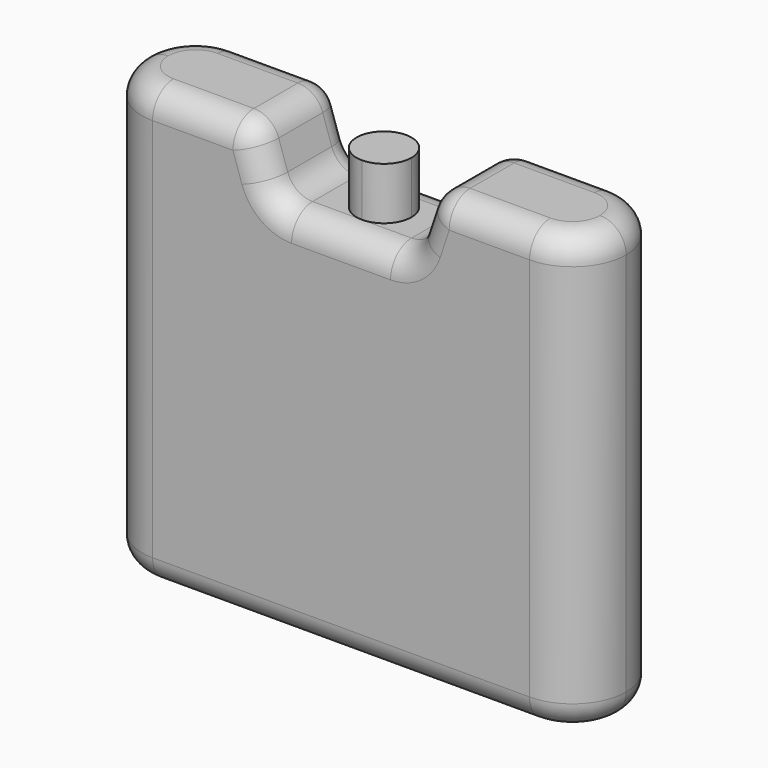
from build123d import *

# Parameters (mm, degrees)
F1_DEPTH = 20.5
F2_R     = 10.24999
F3_F1_R  = 5
F3_F2_R  = 5
F5_DEPTH = 10


# Not quite as in the source:
# - a fillet or chamfer is up to 0.001 mm smaller than in the source, because OpenCascade refuses the exact size


with BuildPart() as f1:
    # F0 (on Front) → F1 (new body)
    with BuildSketch(Plane.XZ):
        Polygon((0, 83.5), (0, 0), (46.25, 0), (46.25, 71.5), (33.2, 71.5), (29.2, 83.5), align=None)
        Polygon((46.25, 71.5), (46.25, 0), (92.5, 0), (92.5, 83.5), (63.3, 83.5), (59.3, 71.5), align=None)
    extrude(amount=F1_DEPTH)

    # F2 (radius 10.25 in the source; OpenCascade refuses exactly that, so slightly less here)
    f2_edges = [f1.edges().sort_by_distance(p)[0] for p in [
        (0, -20.5, 41.75),
        (0, 0, 41.75),
        (92.5, -20.5, 41.75),
        (92.5, 0, 41.75),
    ]]
    fillet(f2_edges, radius=F2_R)

    # F3: fillet of radius 5 on 24 edges, made by hand

    # F3_f1
    f3_f1_edges = [f1.edges().sort_by_distance(p)[0] for p in [
        (59.3, -10.25, 71.5),
        (33.2, -10.25, 71.5),
    ]]
    fillet(f3_f1_edges, radius=F3_F1_R)

    # F3_f2
    f3_f2_edges = [f1.edges().sort_by_distance(p)[0] for p in [
        (92.5, -10.25, 83.5),
        (89.4978474361, -3.0021525639, 83.5),
        (89.4978474361, -17.4978474361, 83.5),
        (72.775005, 0, 83.5),
        (72.775005, -20.5, 83.5),
        (63.3, -10.25, 83.5),
        (0, -10.25, 83.5),
        (3.0021525639, -3.0021525639, 83.5),
        (3.0021525639, -17.4978474361, 83.5),
        (19.724995, 0, 83.5),
        (19.724995, -20.5, 83.5),
        (29.2, -10.25, 83.5),
        (0, -10.25, 0),
        (3.0021525639, -3.0021525639, 0),
        (3.0021525639, -17.4978474361, 0),
        (46.25, 0, 0),
        (46.25, -20.5, 0),
        (89.4978474361, -3.0021525639, 0),
        (89.4978474361, -17.4978474361, 0),
        (92.5, -10.25, 0),
        (46.25, 0, 71.5),
        (46.25, -20.5, 71.5),
        (58.619755323, -20.5, 72.4437890741),
        (33.880244677, -20.5, 72.4437890741),
        (58.619755323, 0, 72.4437890741),
        (33.880244677, 0, 72.4437890741),
    ]]
    fillet(f3_f2_edges, radius=F3_F2_R)

    # F4 (on face) → F5 (join)
    with BuildSketch(Plane.XY.offset(71.5)):
        with BuildLine():
            ThreePointArc((46.25, -15.5), (49.9623106012, -13.9623106012), (51.5, -10.25))
            ThreePointArc((51.5, -10.25), (49.9623106012, -6.5376893988), (46.25, -5))
            ThreePointArc((46.25, -5), (41, -10.25), (46.25, -15.5))
        make_face()
    extrude(amount=F5_DEPTH)


solid = f1.part
